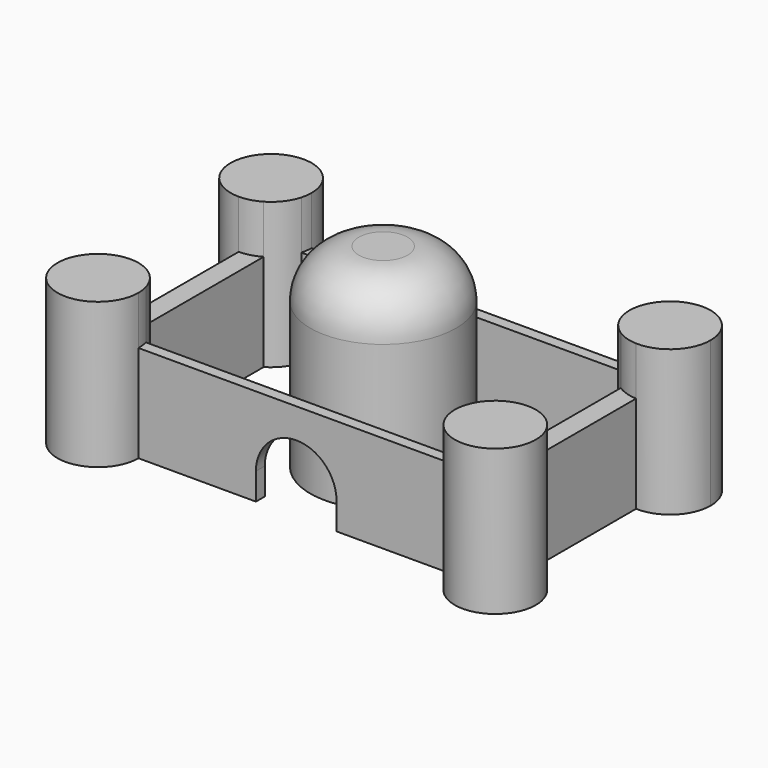
from build123d import *

# Parameters (mm, degrees)
F1_DEPTH = 25.4
F2_DEPTH = 38.1
F0_R     = 19.0813240556
F3_DEPTH = 50.8
F5_DEPTH = 25.4
F6_R     = 12.7


with BuildPart() as f1:
    # F0 (on Top) → F1 (new body)
    with BuildSketch(Plane.XY):
        with BuildLine():
            Line((41.8010411673, 28.3239521086), (-41.3875488453, 28.3239521086))
            ThreePointArc((-41.3875488453, 28.3239521086), (-41.4886521595, 26.8628188405), (-41.7900350118, 25.4295356572))
            Line((-41.7900350118, 25.4295356572), (42.2035273337, 25.4295356572))
            ThreePointArc((42.2035273337, 25.4295356572), (41.9021444815, 26.8628188405), (41.8010411673, 28.3239521086))
        make_face()
    extrude(amount=F1_DEPTH)


with BuildPart() as f1b:
    # F0 (on Top) → F1, piece 2 (new body)
    with BuildSketch(Plane.XY):
        with BuildLine():
            Line((-51.9961640239, 17.7153369301), (-51.9961640239, -17.6895592099))
            ThreePointArc((-51.9961640239, -17.6895592099), (-49.2104219308, -18.0640746947), (-46.6208159924, -19.1570348685))
            Line((-46.6208159924, -19.1570348685), (-46.6208159924, 19.1780049435))
            ThreePointArc((-46.6208159924, 19.1780049435), (-49.2107661987, 18.0875330589), (-51.9961640239, 17.7153369301))
        make_face()
    extrude(amount=F1_DEPTH)


with BuildPart() as f1c:
    # F0 (on Top) → F1, piece 3 (new body)
    with BuildSketch(Plane.XY):
        with BuildLine():
            ThreePointArc((-41.3957258575, -28.2981712371), (-41.3957336891, -28.3110616824), (-41.3957571837, -28.3239521086))
            Line((-41.3957571837, -28.3239521086), (41.3820469809, -28.3239521086))
            ThreePointArc((41.3820469809, -28.3239521086), (41.4827466628, -26.8628475768), (41.7837181231, -25.4295356572))
            Line((41.7837181231, -25.4295356572), (-41.7909358294, -25.4295356572))
            ThreePointArc((-41.7909358294, -25.4295356572), (-41.4949927807, -26.8503054791), (-41.3957258575, -28.2981712371))
        make_face()
    extrude(amount=F1_DEPTH)

    # F4 (on face) → F5 (cut)
    with BuildSketch(Plane.XZ.offset(28.3239521086)):
        with BuildLine():
            Line((-10.6473257765, 7.0293024182), (-10.6473257765, 0))
            Line((-10.6473257765, 0), (10.4405824095, 0))
            Line((10.4405824095, 0), (10.4405824095, 7.0293024182))
            ThreePointArc((10.4405824095, 7.0293024182), (-0.1033716835, 17.5732565112), (-10.6473257765, 7.0293024182))
        make_face()
    extrude(amount=-F5_DEPTH, mode=Mode.SUBTRACT)


with BuildPart() as f1d:
    # F0 (on Top) → F1, piece 4 (new body)
    with BuildSketch(Plane.XY):
        with BuildLine():
            Line((46.6208159924, 19.4339552938), (46.6208159924, -19.1718992682))
            ThreePointArc((46.6208159924, -19.1718992682), (49.210997587, -18.0831005596), (51.9961640239, -17.7124642955))
            Line((51.9961640239, -17.7124642955), (51.9961640239, 17.7233983445))
            ThreePointArc((51.9961640239, 17.7233983445), (49.1927115338, 18.2148481877), (46.6208159924, 19.4339552938))
        make_face()
    extrude(amount=F1_DEPTH)


with BuildPart() as f2:
    # F0 (on Top) → F2 (new body)
    with BuildSketch(Plane.XY):
        with BuildLine():
            ThreePointArc((-41.3875488453, 28.3239521086), (-59.4975877556, 35.8253758404), (-51.9961640239, 17.7153369301))
            ThreePointArc((-51.9961640239, 17.7153369301), (-49.2107661987, 18.0875330589), (-46.6208159924, 19.1780049435))
            ThreePointArc((-46.6208159924, 19.1780049435), (-43.6017601867, 21.8372965586), (-41.7900350118, 25.4295356572))
            ThreePointArc((-41.7900350118, 25.4295356572), (-41.4886521595, 26.8628188405), (-41.3875488453, 28.3239521086))
        make_face()
    extrude(amount=F2_DEPTH)


with BuildPart() as f2b:
    # F0 (on Top) → F2, piece 2 (new body)
    with BuildSketch(Plane.XY):
        with BuildLine():
            ThreePointArc((-51.9961640239, -17.6895592099), (-59.5177610892, -35.7875794321), (-41.3957571837, -28.3239521086))
            ThreePointArc((-41.3957571837, -28.3239521086), (-41.3957336891, -28.3110616824), (-41.3957258575, -28.2981712371))
            ThreePointArc((-41.3957258575, -28.2981712371), (-41.4949927807, -26.8503054791), (-41.7909358294, -25.4295356572))
            ThreePointArc((-41.7909358294, -25.4295356572), (-43.5988592031, -21.8258771182), (-46.6208159924, -19.1570348685))
            ThreePointArc((-46.6208159924, -19.1570348685), (-49.2104219308, -18.0640746947), (-51.9961640239, -17.6895592099))
        make_face()
    extrude(amount=F2_DEPTH)


with BuildPart() as f2c:
    # F0 (on Top) → F2, piece 3 (new body)
    with BuildSketch(Plane.XY):
        with BuildLine():
            ThreePointArc((41.7837181231, -25.4295356572), (41.4827466628, -26.8628475768), (41.3820469809, -28.3239521086))
            ThreePointArc((41.3820469809, -28.3239521086), (51.9920988009, -38.9296931284), (62.5992769487, -28.3210780472))
            ThreePointArc((62.5992769487, -28.3210780472), (59.4940305902, -20.8215999082), (51.9961640239, -17.7124642955))
            ThreePointArc((51.9961640239, -17.7124642955), (49.210997587, -18.0831005596), (46.6208159924, -19.1718992682))
            ThreePointArc((46.6208159924, -19.1718992682), (43.5972956104, -21.8330798569), (41.7837181231, -25.4295356572))
        make_face()
    extrude(amount=F2_DEPTH)


with BuildPart() as f2d:
    # F0 (on Top) → F2, piece 4 (new body)
    with BuildSketch(Plane.XY):
        with BuildLine():
            ThreePointArc((42.2035273337, 25.4295356572), (43.8687836021, 22.0314002589), (46.6208159924, 19.4339552938))
            ThreePointArc((46.6208159924, 19.4339552938), (49.1927115338, 18.2148481877), (51.9961640239, 17.7233983445))
            ThreePointArc((51.9961640239, 17.7233983445), (59.7634354792, 20.6777341896), (63.0182715244, 28.3239521086))
            ThreePointArc((63.0182715244, 28.3239521086), (52.4096563458, 38.9325672872), (41.8010411673, 28.3239521086))
            ThreePointArc((41.8010411673, 28.3239521086), (41.9021444815, 26.8628188405), (42.2035273337, 25.4295356572))
        make_face()
    extrude(amount=F2_DEPTH)


with BuildPart() as f3:
    # F0 (on Top) → F3 (new body)
    with BuildSketch(Plane.XY):
        Circle(F0_R)
    extrude(amount=F3_DEPTH)

    # F6
    f6_edges = [f3.edges().sort_by_distance(p)[0] for p in [
        (-19.081324, 0, 50.8),
    ]]
    fillet(f6_edges, radius=F6_R)


solid = Compound([f1.part, f1b.part, f1c.part, f1d.part, f2.part, f2b.part, f2c.part, f2d.part, f3.part])
